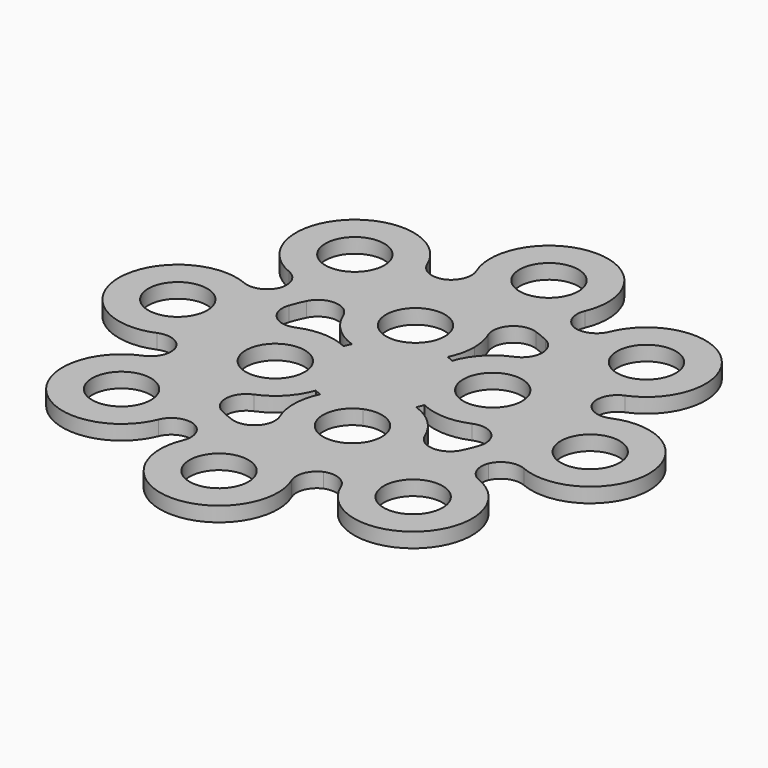
from build123d import *

# Parameters (mm, degrees)
F0_R        = 12.7
F0_R_2      = 6.35
F1_DEPTH    = 3.175
F2_R        = 36.5125
F2_R_2      = 30.1625
F3_DEPTH    = 3.175
F4_T1_DEPTH = 3.175
F6_DEPTH    = 3.175
F7_R        = 4.445


# Not quite as in the source:
# - a fillet or chamfer that OpenCascade refuses, or shapes differently, is made with other operations: its cross-section is extruded or revolved along the edge and cut away or added


with BuildPart() as f1:
    # F0 (on Top) → F1 (new body)
    with BuildSketch(Plane.XY):
        with Locations((44.45, 0)):
            Circle(F0_R)
        with Locations((44.45, 0)):
            Circle(F0_R_2, mode=Mode.SUBTRACT)
    extrude(amount=F1_DEPTH)



with BuildPart() as f1b:
    # F0 (on Top) → F1, piece 2 (new body)
    with BuildSketch(Plane.XY):
        with Locations((31.4308964237, -31.4308964237)):
            Circle(F0_R)
        with Locations((31.4308964237, -31.4308964237)):
            Circle(F0_R_2, mode=Mode.SUBTRACT)
    extrude(amount=F1_DEPTH)


with BuildPart() as f1c:
    # F0 (on Top) → F1, piece 3 (new body)
    with BuildSketch(Plane.XY):
        with Locations((0, -44.45)):
            Circle(F0_R)
        with Locations((0, -44.45)):
            Circle(F0_R_2, mode=Mode.SUBTRACT)
    extrude(amount=F1_DEPTH)


with BuildPart() as f1d:
    # F0 (on Top) → F1, piece 4 (new body)
    with BuildSketch(Plane.XY):
        with Locations((-31.4308964237, -31.4308964237)):
            Circle(F0_R)
        with Locations((-31.4308964237, -31.4308964237)):
            Circle(F0_R_2, mode=Mode.SUBTRACT)
    extrude(amount=F1_DEPTH)


with BuildPart() as f1e:
    # F0 (on Top) → F1, piece 5 (new body)
    with BuildSketch(Plane.XY):
        with Locations((-44.45, 0)):
            Circle(F0_R)
        with Locations((-44.45, 0)):
            Circle(F0_R_2, mode=Mode.SUBTRACT)
    extrude(amount=F1_DEPTH)


with BuildPart() as f1f:
    # F0 (on Top) → F1, piece 6 (new body)
    with BuildSketch(Plane.XY):
        with Locations((-31.4308964237, 31.4308964237)):
            Circle(F0_R)
        with Locations((-31.4308964237, 31.4308964237)):
            Circle(F0_R_2, mode=Mode.SUBTRACT)
    extrude(amount=F1_DEPTH)


with BuildPart() as f1g:
    # F0 (on Top) → F1, piece 7 (new body)
    with BuildSketch(Plane.XY):
        with Locations((0, 44.45)):
            Circle(F0_R)
        with Locations((0, 44.45)):
            Circle(F0_R_2, mode=Mode.SUBTRACT)
    extrude(amount=F1_DEPTH)


with BuildPart() as f1h:
    # F0 (on Top) → F1, piece 8 (new body)
    with BuildSketch(Plane.XY):
        with Locations((31.4308964237, 31.4308964237)):
            Circle(F0_R)
        with Locations((31.4308964237, 31.4308964237)):
            Circle(F0_R_2, mode=Mode.SUBTRACT)
    extrude(amount=F1_DEPTH)


with BuildPart() as f1_1:
    add(f1.part)

    add(f1b.part)  # F3 merges F1b

    add(f1c.part)  # F3 merges F1c

    add(f1d.part)  # F3 merges F1d

    add(f1e.part)  # F3 merges F1e

    add(f1f.part)  # F3 merges F1f

    add(f1g.part)  # F3 merges F1g

    add(f1h.part)  # F3 merges F1h
    # F2 (on Top) → F3 (join)
    with BuildSketch(Plane.XY):
        Circle(F2_R)
        Circle(F2_R_2, mode=Mode.SUBTRACT)
    extrude(amount=F3_DEPTH)

    # F4: fillet of radius 4.445 on 16 edges, made by hand

    # F4_s2 → F4_t1 (join)
    with BuildSketch(Plane.XY):
        with BuildLine():
            ThreePointArc((13.8619814715, -33.7788117899), (17.2703456097, -33.7926240048), (19.6669191039, -36.2161694167))
            ThreePointArc((19.6669191039, -36.2161694167), (18.9586174739, -33.8251098221), (18.7312093993, -31.3417365615))
            ThreePointArc((18.7312093993, -31.3417365615), (16.3420885049, -32.6511684255), (13.8619814715, -33.7788117899))
        make_face()
        with BuildLine():
            ThreePointArc((36.2161694167, -19.6669191039), (33.7926240048, -17.2703456097), (33.7788117899, -13.8619814715))
            ThreePointArc((33.7788117899, -13.8619814715), (32.6511684255, -16.3420885049), (31.3417365615, -18.7312093993))
            ThreePointArc((31.3417365615, -18.7312093993), (33.8251098221, -18.9586174739), (36.2161694167, -19.6669191039))
        make_face()
        with BuildLine():
            ThreePointArc((-14.0833257779, -33.6871279762), (-11.6830150938, -36.106972082), (-11.7020871198, -39.5153108466))
            ThreePointArc((-11.7020871198, -39.5153108466), (-10.5121975519, -37.3237315073), (-8.9169892707, -35.4069196429))
            ThreePointArc((-8.9169892707, -35.4069196429), (-11.5322610068, -34.6434642079), (-14.0833257779, -33.6871279762))
        make_face()
        with BuildLine():
            ThreePointArc((11.7020871198, -39.5153108466), (11.6830150938, -36.106972082), (14.0833257779, -33.6871279762))
            ThreePointArc((14.0833257779, -33.6871279762), (11.5322610068, -34.6434642079), (8.9169892707, -35.4069196429))
            ThreePointArc((8.9169892707, -35.4069196429), (10.5121975519, -37.3237315073), (11.7020871198, -39.5153108466))
        make_face()
        with BuildLine():
            ThreePointArc((33.6871279762, -14.0833257779), (36.106972082, -11.6830150938), (39.5153108466, -11.7020871198))
            ThreePointArc((39.5153108466, -11.7020871198), (37.3237315073, -10.5121975519), (35.4069196429, -8.9169892707))
            ThreePointArc((35.4069196429, -8.9169892707), (34.6434642079, -11.5322610068), (33.6871279762, -14.0833257779))
        make_face()
        with BuildLine():
            ThreePointArc((39.5153108466, 11.7020871198), (36.106972082, 11.6830150938), (33.6871279762, 14.0833257779))
            ThreePointArc((33.6871279762, 14.0833257779), (34.6434642079, 11.5322610068), (35.4069196429, 8.9169892707))
            ThreePointArc((35.4069196429, 8.9169892707), (37.3237315073, 10.5121975519), (39.5153108466, 11.7020871198))
        make_face()
        with BuildLine():
            ThreePointArc((36.2161694167, 19.6669191039), (33.7926240048, 17.2703456097), (33.7788117899, 13.8619814715))
            ThreePointArc((33.7788117899, 13.8619814715), (32.6511684255, 16.3420885049), (31.3417365615, 18.7312093993))
            ThreePointArc((31.3417365615, 18.7312093993), (33.8251098221, 18.9586174739), (36.2161694167, 19.6669191039))
        make_face()
        with BuildLine():
            ThreePointArc((19.6669191039, 36.2161694167), (17.2703456097, 33.7926240048), (13.8619814715, 33.7788117899))
            ThreePointArc((13.8619814715, 33.7788117899), (16.3420885049, 32.6511684255), (18.7312093993, 31.3417365615))
            ThreePointArc((18.7312093993, 31.3417365615), (18.9586174739, 33.8251098221), (19.6669191039, 36.2161694167))
        make_face()
        with BuildLine():
            ThreePointArc((14.0833257779, 33.6871279762), (11.6830150938, 36.106972082), (11.7020871198, 39.5153108466))
            ThreePointArc((11.7020871198, 39.5153108466), (10.5121975519, 37.3237315073), (8.9169892707, 35.4069196429))
            ThreePointArc((8.9169892707, 35.4069196429), (11.5322610068, 34.6434642079), (14.0833257779, 33.6871279762))
        make_face()
        with BuildLine():
            ThreePointArc((-11.7020871198, 39.5153108466), (-11.6830150938, 36.106972082), (-14.0833257779, 33.6871279762))
            ThreePointArc((-14.0833257779, 33.6871279762), (-11.5322610068, 34.6434642079), (-8.9169892707, 35.4069196429))
            ThreePointArc((-8.9169892707, 35.4069196429), (-10.5121975519, 37.3237315073), (-11.7020871198, 39.5153108466))
        make_face()
        with BuildLine():
            ThreePointArc((-13.8619814715, 33.7788117899), (-17.2703456097, 33.7926240048), (-19.6669191039, 36.2161694167))
            ThreePointArc((-19.6669191039, 36.2161694167), (-18.9586174739, 33.8251098221), (-18.7312093993, 31.3417365615))
            ThreePointArc((-18.7312093993, 31.3417365615), (-16.3420885049, 32.6511684255), (-13.8619814715, 33.7788117899))
        make_face()
        with BuildLine():
            ThreePointArc((-36.2161694167, 19.6669191039), (-33.7926240048, 17.2703456097), (-33.7788117899, 13.8619814715))
            ThreePointArc((-33.7788117899, 13.8619814715), (-32.6511684255, 16.3420885049), (-31.3417365615, 18.7312093993))
            ThreePointArc((-31.3417365615, 18.7312093993), (-33.8251098221, 18.9586174739), (-36.2161694167, 19.6669191039))
        make_face()
        with BuildLine():
            ThreePointArc((-39.5153108466, -11.7020871198), (-36.106972082, -11.6830150938), (-33.6871279762, -14.0833257779))
            ThreePointArc((-33.6871279762, -14.0833257779), (-34.6434642079, -11.5322610068), (-35.4069196429, -8.9169892707))
            ThreePointArc((-35.4069196429, -8.9169892707), (-37.3237315073, -10.5121975519), (-39.5153108466, -11.7020871198))
        make_face()
        with BuildLine():
            ThreePointArc((-33.6871279762, 14.0833257779), (-36.106972082, 11.6830150938), (-39.5153108466, 11.7020871198))
            ThreePointArc((-39.5153108466, 11.7020871198), (-37.3237315073, 10.5121975519), (-35.4069196429, 8.9169892707))
            ThreePointArc((-35.4069196429, 8.9169892707), (-34.6434642079, 11.5322610068), (-33.6871279762, 14.0833257779))
        make_face()
        with BuildLine():
            ThreePointArc((-33.7788117899, -13.8619814715), (-33.7926240048, -17.2703456097), (-36.2161694167, -19.6669191039))
            ThreePointArc((-36.2161694167, -19.6669191039), (-33.8251098221, -18.9586174739), (-31.3417365615, -18.7312093993))
            ThreePointArc((-31.3417365615, -18.7312093993), (-32.6511684255, -16.3420885049), (-33.7788117899, -13.8619814715))
        make_face()
        with BuildLine():
            ThreePointArc((-19.6669191039, -36.2161694167), (-17.2703456097, -33.7926240048), (-13.8619814715, -33.7788117899))
            ThreePointArc((-13.8619814715, -33.7788117899), (-16.3420885049, -32.6511684255), (-18.7312093993, -31.3417365615))
            ThreePointArc((-18.7312093993, -31.3417365615), (-18.9586174739, -33.8251098221), (-19.6669191039, -36.2161694167))
        make_face()
    extrude(amount=F4_T1_DEPTH)

    # F5 (on Top) → F6 (join)
    with BuildSketch(Plane.XY):
        with BuildLine():
            ThreePointArc((-4.8600797817, 11.7332699839), (-0.3978508652, 12.6937667652), (4.1157689697, 12.0145930346))
            ThreePointArc((4.1157689697, 12.0145930346), (5.0821233795, 14.7332678767), (5.4098806134, 17.5999050943))
            ThreePointArc((5.4098806134, 17.5999050943), (-14.6731991669, 27.9333523874), (-11.4058883563, 5.5853120597))
            ThreePointArc((-11.4058883563, 5.5853120597), (-8.6945256642, 9.2571714619), (-4.8600797817, 11.7332699839))
        make_face()
        with BuildLine():
            ThreePointArc((-0.9401193866, 17.5999050943), (-2.0102874057, 14.0720340289), (-4.8600797817, 11.7332699839))
            ThreePointArc((-4.8600797817, 11.7332699839), (-12.5699513674, 21.1277761598), (-0.9401193866, 17.5999050943))
        make_face(mode=Mode.SUBTRACT)
        with BuildLine():
            ThreePointArc((-11.7332700028, -4.860079736), (-12.693766766, -0.3978508405), (-12.0145930346, 4.1157689697))
            ThreePointArc((-12.0145930346, 4.1157689697), (-29.3331751572, -12.1501989776), (-5.5853120597, -11.4058883563))
            ThreePointArc((-5.5853120597, -11.4058883563), (-9.2571714788, -8.6945256462), (-11.7332700028, -4.860079736))
        make_face()
        with BuildLine():
            ThreePointArc((-11.2499050943, -7.2901193866), (-23.8278916402, -8.5289428544), (-11.7332700028, -4.860079736))
            ThreePointArc((-11.7332700028, -4.860079736), (-11.3719185485, -6.0512959187), (-11.2499050943, -7.2901193866))
        make_face(mode=Mode.SUBTRACT)
        with BuildLine():
            ThreePointArc((19.9901193866, -17.5999050943), (17.6235666796, -10.216825314), (11.4058883563, -5.5853120597))
            ThreePointArc((11.4058883563, -5.5853120597), (8.6945256544, -9.2571714711), (4.8600797567, -11.7332699943))
            ThreePointArc((4.8600797567, -11.7332699943), (0.3978508516, -12.6937667656), (-4.1157689697, -12.0145930346))
            ThreePointArc((-4.1157689697, -12.0145930346), (4.4234821689, -29.9721478604), (19.9901193866, -17.5999050943))
        make_face()
        with BuildLine():
            ThreePointArc((13.6401193866, -17.5999050943), (3.7622483323, -22.8797370827), (4.8600797567, -11.7332699943))
            ThreePointArc((4.8600797567, -11.7332699943), (10.8179904408, -12.320073106), (13.6401193866, -17.5999050943))
        make_face(mode=Mode.SUBTRACT)
        with BuildLine():
            ThreePointArc((12.0145930346, -4.1157689697), (24.3213832369, -3.4853959876), (30.2999050943, 7.2901193866))
            ThreePointArc((30.2999050943, 7.2901193866), (19.6861299696, 19.8175958192), (5.5853120597, 11.4058883563))
            ThreePointArc((5.5853120597, 11.4058883563), (9.2571714786, 8.6945256464), (11.7332700027, 4.8600797365))
            ThreePointArc((11.7332700027, 4.8600797365), (12.4559730458, 2.4776471668), (12.7, 0))
            ThreePointArc((12.7, 0), (12.5274764326, -2.0862248752), (12.0145930346, -4.1157689697))
        make_face()
        with BuildLine():
            ThreePointArc((23.9499050943, 7.2901193866), (18.8387285619, 1.0621328406), (11.7332700027, 4.8600797365))
            ThreePointArc((11.7332700027, 4.8600797365), (16.3610816267, 13.5181059325), (23.9499050943, 7.2901193866))
        make_face(mode=Mode.SUBTRACT)
        with BuildLine():
            ThreePointArc((12.0145930346, -4.1157689697), (5.8666350314, 2.4300397955), (5.5853120597, 11.4058883563))
            ThreePointArc((5.5853120597, 11.4058883563), (4.860079591, 11.7332700629), (4.1157689697, 12.0145930346))
            ThreePointArc((4.1157689697, 12.0145930346), (-2.4300397955, 5.8666350314), (-11.4058883563, 5.5853120597))
            ThreePointArc((-11.4058883563, 5.5853120597), (-11.7332700629, 4.860079591), (-12.0145930346, 4.1157689697))
            ThreePointArc((-12.0145930346, 4.1157689697), (-6.8243897202, -0.568641244), (-4.8999050943, -7.2901193866))
            ThreePointArc((-4.8999050943, -7.2901193866), (-5.0724286617, -9.3763442618), (-5.5853120597, -11.4058883563))
            ThreePointArc((-5.5853120597, -11.4058883563), (-4.860079591, -11.7332700629), (-4.1157689697, -12.0145930346))
            ThreePointArc((-4.1157689697, -12.0145930346), (2.4300397955, -5.8666350314), (11.4058883563, -5.5853120597))
            ThreePointArc((11.4058883563, -5.5853120597), (11.7332700629, -4.860079591), (12.0145930346, -4.1157689697))
        make_face()
        with BuildLine():
            ThreePointArc((-4.8999050943, -7.2901193866), (-6.8243897202, -0.568641244), (-12.0145930346, 4.1157689697))
            ThreePointArc((-12.0145930346, 4.1157689697), (-12.693766766, -0.3978508405), (-11.7332700028, -4.860079736))
            ThreePointArc((-11.7332700028, -4.860079736), (-9.2571714788, -8.6945256462), (-5.5853120597, -11.4058883563))
            ThreePointArc((-5.5853120597, -11.4058883563), (-5.0724286617, -9.3763442618), (-4.8999050943, -7.2901193866))
        make_face()
        with BuildLine():
            ThreePointArc((-11.4058883563, 5.5853120597), (-2.4300397955, 5.8666350314), (4.1157689697, 12.0145930346))
            ThreePointArc((4.1157689697, 12.0145930346), (-0.3978508652, 12.6937667652), (-4.8600797817, 11.7332699839))
            ThreePointArc((-4.8600797817, 11.7332699839), (-8.6945256642, 9.2571714619), (-11.4058883563, 5.5853120597))
        make_face()
        with BuildLine():
            ThreePointArc((11.7332700027, 4.8600797365), (9.2571714786, 8.6945256464), (5.5853120597, 11.4058883563))
            ThreePointArc((5.5853120597, 11.4058883563), (5.8666350314, 2.4300397955), (12.0145930346, -4.1157689697))
            ThreePointArc((12.0145930346, -4.1157689697), (12.5274764326, -2.0862248752), (12.7, 0))
            ThreePointArc((12.7, 0), (12.4559730458, 2.4776471668), (11.7332700027, 4.8600797365))
        make_face()
        with BuildLine():
            ThreePointArc((4.8600797567, -11.7332699943), (8.6945256544, -9.2571714711), (11.4058883563, -5.5853120597))
            ThreePointArc((11.4058883563, -5.5853120597), (2.4300397955, -5.8666350314), (-4.1157689697, -12.0145930346))
            ThreePointArc((-4.1157689697, -12.0145930346), (0.3978508516, -12.6937667656), (4.8600797567, -11.7332699943))
        make_face()
    extrude(amount=F6_DEPTH)

    # F7
    f7_edges = [f1_1.edges().sort_by_distance(p)[0] for p in [
        (-18.251583, 24.013666, 1.5875),
        (-4.074408, 29.886044, 1.5875),
        (-24.013666, -18.251583, 1.5875),
        (-29.886044, -4.074408, 1.5875),
        (24.013666, 18.251583, 1.5875),
        (29.886044, 4.074408, 1.5875),
        (4.074408, -29.886044, 1.5875),
        (18.251583, -24.013666, 1.5875),
    ]]
    fillet(f7_edges, radius=F7_R)


solid = f1_1.part
